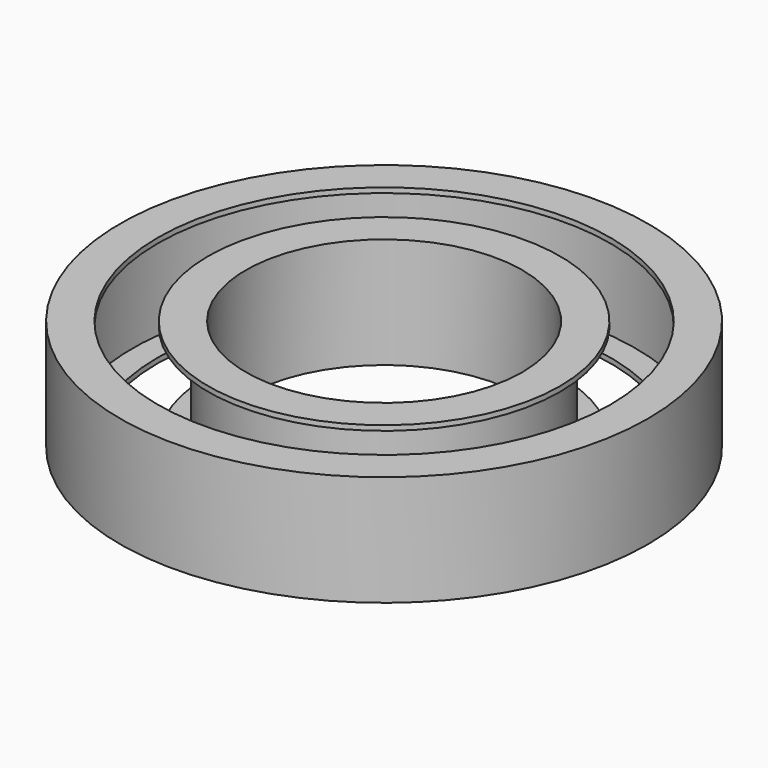
from build123d import *

# Parameters (mm, degrees)
F0_R      = 5.25
F0_R_2    = 5
F1_DEPTH  = 2
F0_R_3    = 3
F0_R_4    = 2.75
F7_R      = 5.25
F7_R_2    = 5
F7_R_3    = 4.4998566685
F8_DEPTH  = 0.1
F7_R_4    = 3.5
F7_R_5    = 3
F7_R_6    = 2.75
F9_R      = 3.5
F9_R_2    = 3
F9_R_3    = 2.75
F10_DEPTH = 0.1
F9_R_4    = 5.25
F9_R_5    = 4.5


# Not quite as in the source:
# - a feature of the source that left no trace in its solid (it failed there, or was rolled back) is left out
# - the program builds the solid bodies; features that only make, move or delete a surface that nothing else refers to are left out


with BuildPart() as f1:
    # F0 (on Top) → F1 (new body)
    with BuildSketch(Plane.XY):
        Circle(F0_R)
        Circle(F0_R_2, mode=Mode.SUBTRACT)
    extrude(amount=F1_DEPTH)

    # F7 (on face) → F8 (join)
    with BuildSketch(Plane.XY.offset(2)):
        Circle(F7_R)
        Circle(F7_R_2, mode=Mode.SUBTRACT)
        Circle(F7_R_2)
        Circle(F7_R_3, mode=Mode.SUBTRACT)
    extrude(amount=F8_DEPTH)

    # F9 (on face) → F10, piece 2 (join)
    with BuildSketch(Plane(origin=(0, 0, 0), x_dir=(1, 0, 0), z_dir=(0, 0, -1))):
        Circle(F9_R_4)
        Circle(F9_R_5, mode=Mode.SUBTRACT)
    extrude(amount=F10_DEPTH)


with BuildPart() as f1b:
    # F0 (on Top) → F1, piece 2 (new body)
    with BuildSketch(Plane.XY):
        Circle(F0_R_3)
        Circle(F0_R_4, mode=Mode.SUBTRACT)
    extrude(amount=F1_DEPTH)

    # F7 (on face) → F8, piece 2 (join)
    with BuildSketch(Plane.XY.offset(2)):
        Circle(F7_R_4)
        Circle(F7_R_5, mode=Mode.SUBTRACT)
        Circle(F7_R_5)
        Circle(F7_R_6, mode=Mode.SUBTRACT)
    extrude(amount=F8_DEPTH)

    # F9 (on face) → F10 (join)
    with BuildSketch(Plane(origin=(0, 0, 0), x_dir=(1, 0, 0), z_dir=(0, 0, -1))):
        Circle(F9_R)
        Circle(F9_R_2, mode=Mode.SUBTRACT)
        Circle(F9_R_2)
        Circle(F9_R_3, mode=Mode.SUBTRACT)
    extrude(amount=F10_DEPTH)


solid = Compound([f1.part, f1b.part])
